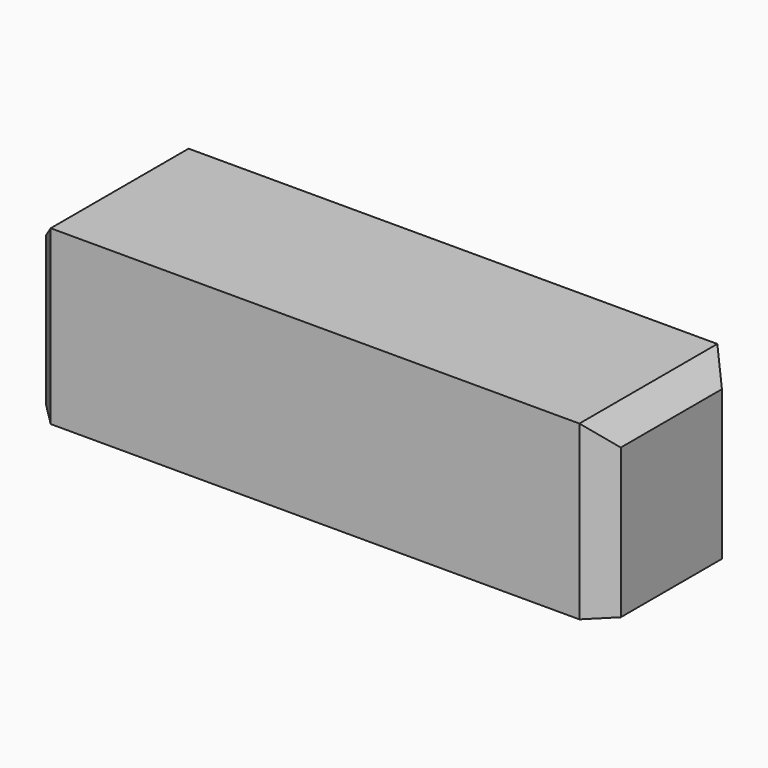
from build123d import *

# Parameters (mm, degrees)
F0_W     = 10
F0_H     = 3
F1_DEPTH = 3
F3_SIZE  = 0.4


# Not quite as in the source:
# - a feature of the source that left no trace in its solid (it failed there, or was rolled back) is left out


with BuildPart() as f1:
    # F0 (on Top) → F1 (new body)
    with BuildSketch(Plane.XY):
        Rectangle(F0_W, F0_H)
    extrude(amount=F1_DEPTH)

    # F3
    f3_edges = [f1.edges().sort_by_distance(p)[0] for p in [
        (5, -1.5, 1.5),
        (5, 1.5, 1.5),
        (-5, -1.5, 1.5),
        (-5, 1.5, 1.5),
        (5, 0, 3),
        (-5, 0, 3),
    ]]
    chamfer(f3_edges, length=F3_SIZE)


solid = f1.part
